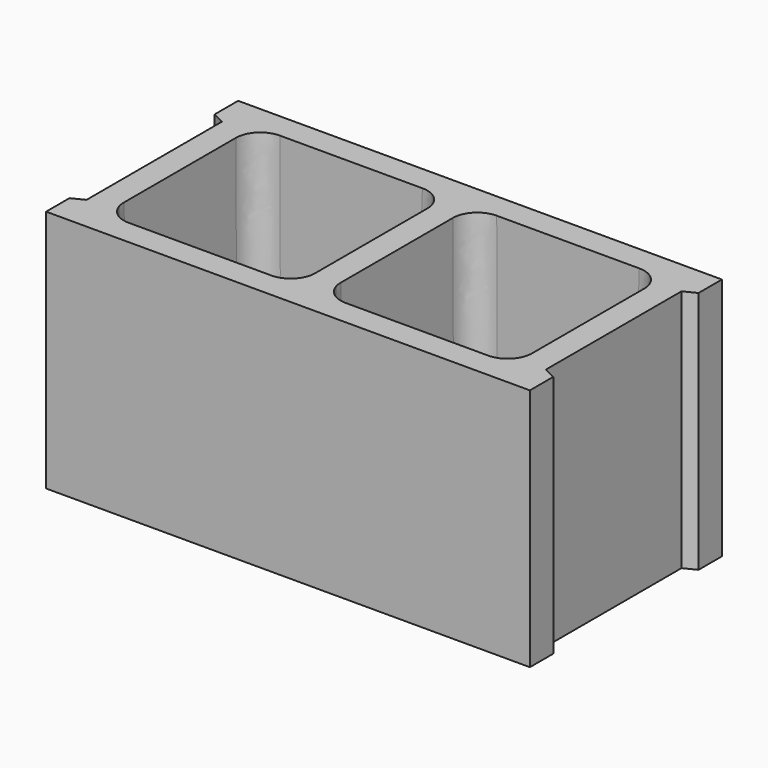
from build123d import *

# Parameters (mm, degrees)
F0_W          = 198.5
F0_H          = 197
F1_DEPTH      = 200
F2_W          = 157
F2_H          = 155
F3_DEPTH      = 158
F3_TAPER      = 1.1
F3_FACE_W     = 150.9324900332
F3_FACE_H     = 148.9324900332
F4_DEPTH      = 42.001
F4_TAPER      = 18.5
F5_W          = 10
F5_H          = 149
F6_DEPTH      = 200.0010001
F8_F1_R       = 20
F8_F2_R       = 20
F8_F3_R       = 20
F8_F4_R       = 20
F9_F1_R       = 20
F9_F2_R       = 20
F9_F3_R       = 20
F9_F4_R       = 20
F10_F1_R      = 20
F10_F2_R      = 20
F11_F1_R      = 20
F11_F2_R      = 20
F12_F1_R      = 20
F12_F2_R      = 20
F12_F3_R      = 20
F12_F4_R      = 20
F13_T4_DEPTH  = 200
F13_T9_DEPTH  = 200
F13_T14_DEPTH = 200
F13_T19_DEPTH = 200


# Not quite as in the source:
# - a fillet or chamfer that OpenCascade refuses, or shapes differently, is made with other operations: its cross-section is extruded or revolved along the edge and cut away or added
# - two fillets or chamfers of one size are made in one step


with BuildPart() as f1:
    # F0 (on Top) → F1 (new body)
    with BuildSketch(Plane.XY):
        with Locations((-99.25, 0)):
            Rectangle(F0_W, F0_H)
    extrude(amount=F1_DEPTH)

    # F2 (on face) → F3 (cut)
    with BuildSketch(Plane.XY.offset(200)):
        with Locations((-89, 0)):
            Rectangle(F2_W, F2_H)
    extrude(amount=-F3_DEPTH, taper=F3_TAPER, mode=Mode.SUBTRACT)

    # F3_face (on face) → F4 (cut, through all)
    with BuildSketch(Plane(origin=(-89, 0, 42), x_dir=(1, 0, 0), z_dir=(0, 0, 1))):
        Rectangle(F3_FACE_W, F3_FACE_H)
    extrude(amount=-F4_DEPTH, taper=F4_TAPER, mode=Mode.SUBTRACT)

    # F5 (on face) → F6 (cut, through all)
    with BuildSketch(Plane.XY.offset(200)):
        with Locations((-193.5, 0)):
            Rectangle(F5_W, F5_H)
    extrude(amount=-F6_DEPTH, mode=Mode.SUBTRACT)

    # F7: F1 across plane


with BuildPart() as f1_1:
    add(f1.part)
    add(f1.part.mirror(Plane.YZ))

    # F8: fillet of radius 20 on 4 edges, made by hand

    # F8_f1
    f8_f1_edges = [f1_1.edges().sort_by_distance(p)[0] for p in [
        (157.439743307, -67.439743307, 21),
    ]]
    fillet(f8_f1_edges, radius=F8_F1_R)

    # F8_f2
    f8_f2_edges = [f1_1.edges().sort_by_distance(p)[0] for p in [
        (-20.560256693, -67.439743307, 21),
    ]]
    fillet(f8_f2_edges, radius=F8_F2_R)

    # F8_f3
    f8_f3_edges = [f1_1.edges().sort_by_distance(p)[0] for p in [
        (166.1488465087, -76.1488465087, 129.6310174042),
    ]]
    fillet(f8_f3_edges, radius=F8_F3_R)

    # F8_f4
    f8_f4_edges = [f1_1.edges().sort_by_distance(p)[0] for p in [
        (-11.8511534913, -76.1488465087, 129.6310174042),
    ]]
    fillet(f8_f4_edges, radius=F8_F4_R)

    # F9: fillet of radius 20 on 4 edges, made by hand

    # F9_f1
    f9_f1_edges = [f1_1.edges().sort_by_distance(p)[0] for p in [
        (-157.439743307, -67.439743307, 21),
    ]]
    fillet(f9_f1_edges, radius=F9_F1_R)

    # F9_f2
    f9_f2_edges = [f1_1.edges().sort_by_distance(p)[0] for p in [
        (20.560256693, -67.439743307, 21),
    ]]
    fillet(f9_f2_edges, radius=F9_F2_R)

    # F9_f3
    f9_f3_edges = [f1_1.edges().sort_by_distance(p)[0] for p in [
        (-166.1488465087, -76.1488465087, 129.6310174042),
    ]]
    fillet(f9_f3_edges, radius=F9_F3_R)

    # F9_f4
    f9_f4_edges = [f1_1.edges().sort_by_distance(p)[0] for p in [
        (11.8511534913, -76.1488465087, 129.6310174042),
    ]]
    fillet(f9_f4_edges, radius=F9_F4_R)

    # F10: fillet of radius 20 on 2 edges, made by hand

    # F10_f1
    f10_f1_edges = [f1_1.edges().sort_by_distance(p)[0] for p in [
        (-157.439743307, 67.439743307, 21),
    ]]
    fillet(f10_f1_edges, radius=F10_F1_R)

    # F10_f2
    f10_f2_edges = [f1_1.edges().sort_by_distance(p)[0] for p in [
        (-166.1488465087, 76.1488465087, 129.6310174042),
    ]]
    fillet(f10_f2_edges, radius=F10_F2_R)

    # F11: fillet of radius 20 on 2 edges, made by hand

    # F11_f1
    f11_f1_edges = [f1_1.edges().sort_by_distance(p)[0] for p in [
        (20.560256693, 67.439743307, 21),
    ]]
    fillet(f11_f1_edges, radius=F11_F1_R)

    # F11_f2
    f11_f2_edges = [f1_1.edges().sort_by_distance(p)[0] for p in [
        (11.8511534913, 76.1488465087, 129.6310174042),
    ]]
    fillet(f11_f2_edges, radius=F11_F2_R)

    # F12: fillet of radius 20 on 4 edges, made by hand

    # F12_f1
    f12_f1_edges = [f1_1.edges().sort_by_distance(p)[0] for p in [
        (157.439743307, 67.439743307, 21),
    ]]
    fillet(f12_f1_edges, radius=F12_F1_R)

    # F12_f2
    f12_f2_edges = [f1_1.edges().sort_by_distance(p)[0] for p in [
        (-20.560256693, 67.439743307, 21),
    ]]
    fillet(f12_f2_edges, radius=F12_F2_R)

    # F12_f3
    f12_f3_edges = [f1_1.edges().sort_by_distance(p)[0] for p in [
        (166.1488465087, 76.1488465087, 129.6310174042),
    ]]
    fillet(f12_f3_edges, radius=F12_F3_R)

    # F12_f4
    f12_f4_edges = [f1_1.edges().sort_by_distance(p)[0] for p in [
        (-11.8511534913, 76.1488465087, 129.6310174042),
    ]]
    fillet(f12_f4_edges, radius=F12_F4_R)

    # F13: chamfer of 5 x 10 on 4 edges, made by hand


with BuildPart() as f13_tool2:
    # F13_s3 → F13_t4 (new body)
    with BuildSketch(Plane.XY.offset(200)):
        Polygon((188.5, 69.5), (198.5, 74.5), (188.5, 74.5), align=None)
    extrude(amount=-F13_T4_DEPTH)

    split(bisect_by=Plane.YZ.offset(198.5), keep=Keep.BOTTOM)


with BuildPart() as f1_2:
    add(f1_1.part)

    # F13_t1: union F13_tool2
    add(f13_tool2.part)


with BuildPart() as f13_tool7:
    # F13_s8 → F13_t9 (new body)
    with BuildSketch(Plane.XY.offset(200)):
        Polygon((198.5, -74.5), (188.5, -69.5), (188.5, -74.5), align=None)
    extrude(amount=-F13_T9_DEPTH)

    split(bisect_by=Plane.YZ.offset(198.5), keep=Keep.BOTTOM)


with BuildPart() as f1_3:
    add(f1_2.part)

    # F13_t6: union F13_tool7
    add(f13_tool7.part)


with BuildPart() as f13_tool12:
    # F13_s13 → F13_t14 (new body)
    with BuildSketch(Plane.XY.offset(200)):
        Polygon((-198.5, 74.5), (-188.5, 69.5), (-188.5, 74.5), align=None)
    extrude(amount=-F13_T14_DEPTH)

    split(bisect_by=Plane.YZ.offset(-198.5), keep=Keep.TOP)


with BuildPart() as f1_4:
    add(f1_3.part)

    # F13_t11: union F13_tool12
    add(f13_tool12.part)


with BuildPart() as f13_tool17:
    # F13_s18 → F13_t19 (new body)
    with BuildSketch(Plane.XY.offset(200)):
        Polygon((-188.5, -69.5), (-198.5, -74.5), (-188.5, -74.5), align=None)
    extrude(amount=-F13_T19_DEPTH)

    split(bisect_by=Plane.YZ.offset(-198.5), keep=Keep.TOP)


with BuildPart() as f1_5:
    add(f1_4.part)

    # F13_t16: union F13_tool17
    add(f13_tool17.part)


with BuildPart() as f15_1:
    # F15: copy of F1
    add(f1_5.part)


solid = f1_5.part
